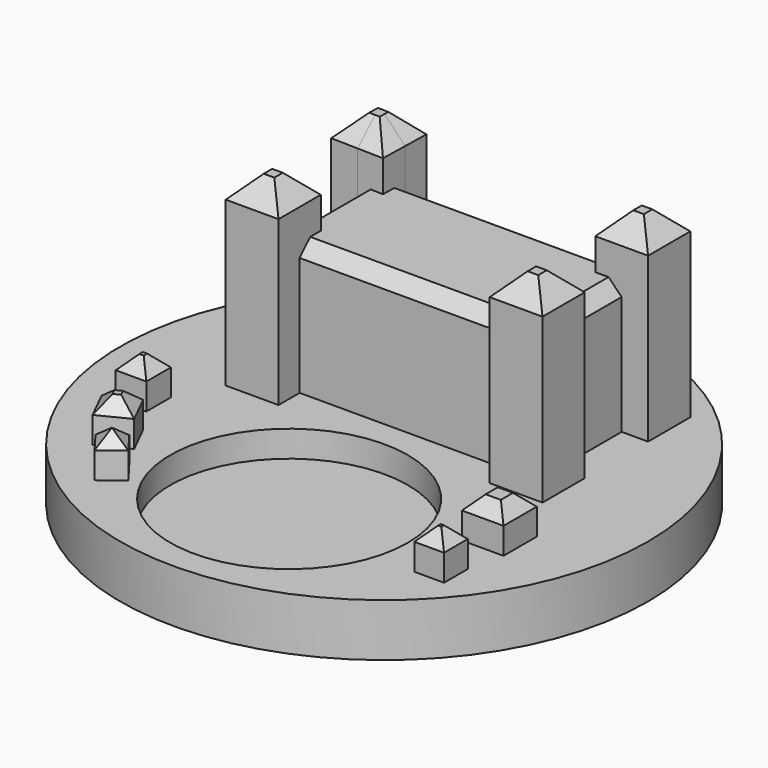
from build123d import *

# Parameters (mm, degrees)
F0_R     = 25.4
F0_W     = 2.9527507722
F0_H     = 2.9527507722
F0_R_2   = 11.43
F0_W_2   = 2.8575006872
F0_H_2   = 2.8575006872
F0_W_3   = 4.0005007759
F0_H_3   = 4.0005007759
F1_DEPTH = 5.08
F2_DEPTH = 2.54
F3_DEPTH = 17.78
F0_W_4   = 2.54
F0_H_4   = 2.54
F0_W_5   = 2.5392780889
F0_H_5   = 2.5392780889
F4_DEPTH = 22.86
F5_DEPTH = 8.89
F6_SIZE  = 1.26999
F7_SIZE  = 2.032
F8_SIZE  = 1.27


# Not quite as in the source:
# - a fillet or chamfer is up to 0.001 mm smaller than in the source, because OpenCascade refuses the exact size


with BuildPart() as f1:
    # F0 (on Top) → F1 (new body)
    with BuildSketch(Plane.XY):
        Circle(F0_R)
        Polygon((-14.8460203377, -16.160586299), (-12.8199555069, -14.6287046778), (-11.2880738857, -16.6547695086), (-13.3141387165, -18.1866511298), align=None, mode=Mode.SUBTRACT)
        Polygon((-17.0199228451, -13.7883033603), (-18.4486722574, -10.9308026731), (-15.5911715701, -9.5020532608), (-14.1624221578, -12.359553948), align=None, mode=Mode.SUBTRACT)
        with Locations((-18.734421581, -5.5491779931)):
            Rectangle(F0_W, F0_H, mode=Mode.SUBTRACT)
        with Locations((0, -11.43)):
            Circle(F0_R_2, mode=Mode.SUBTRACT)
        with Locations((16.1819914356, -13.3789330721)):
            Rectangle(F0_W_2, F0_H_2, mode=Mode.SUBTRACT)
        with Locations((16.3652040064, -6.5969279967)):
            Rectangle(F0_W_3, F0_H_3, mode=Mode.SUBTRACT)
        Polygon((-10.1001541496, 17.7187103274), (-10.1592772274, 15.24), (10.1607219111, 15.24), (10.1607219111, 17.7792780889), (15.2392780889, 17.7792780889), (15.2392780889, 12.7007219111), (12.7, 12.7007219111), (12.7, 5.08), (15.24, 5.08), (15.24, 0), (10.16, 0), (10.16, 2.54), (-10.16, 2.54), (-10.16, 0), (-15.24, 0), (-15.24, 5.08), (-12.7, 5.08), (-12.7, 12.6992772274), (-15.2998458504, 12.7612896726), (-15.1787103274, 17.8398458504), align=None, mode=Mode.SUBTRACT)
    extrude(amount=F1_DEPTH)

    # F0 (on Top) → F2 (join)
    with BuildSketch(Plane.XY):
        with Locations((0, -11.43)):
            Circle(F0_R_2)
    extrude(amount=F2_DEPTH)

    # F0 (on Top) → F3 (join)
    with BuildSketch(Plane.XY):
        Polygon((10.1607219111, 15.24), (-10.1592772274, 15.24), (-10.2212896726, 12.6401541496), (-12.7, 12.6992772274), (-12.7, 5.08), (-10.16, 5.08), (-10.16, 2.54), (10.16, 2.54), (10.16, 5.08), (12.7, 5.08), (12.7, 12.7007219111), (10.1607219111, 12.7007219111), align=None)
    extrude(amount=F3_DEPTH)

    # F0 (on Top) → F4 (join)
    with BuildSketch(Plane.XY):
        Polygon((-10.1592772274, 15.24), (-12.7, 15.24), (-12.7, 12.6992772274), (-10.2212896726, 12.6401541496), align=None)
        Polygon((-12.7, 12.6992772274), (-12.7, 15.24), (-10.1592772274, 15.24), (-10.1001541496, 17.7187103274), (-15.1787103274, 17.8398458504), (-15.2998458504, 12.7612896726), align=None)
        with Locations((-11.43, 3.81)):
            Rectangle(F0_W_4, F0_H_4)
        Polygon((-12.7, 2.54), (-12.7, 5.08), (-15.24, 5.08), (-15.24, 0), (-10.16, 0), (-10.16, 2.54), align=None)
        with Locations((11.4303609556, 13.9703609556)):
            Rectangle(F0_W_5, F0_H_5)
        Polygon((10.1607219111, 17.7792780889), (10.1607219111, 15.24), (12.7, 15.24), (12.7, 12.7007219111), (15.2392780889, 12.7007219111), (15.2392780889, 17.7792780889), align=None)
        with Locations((11.43, 3.81)):
            Rectangle(F0_W_4, F0_H_4)
        Polygon((15.24, 5.08), (12.7, 5.08), (12.7, 2.54), (10.16, 2.54), (10.16, 0), (15.24, 0), align=None)
    extrude(amount=F4_DEPTH)

    # F0 (on Top) → F5 (join)
    with BuildSketch(Plane.XY):
        with Locations((-18.734421581, -5.5491779931)):
            Rectangle(F0_W, F0_H)
        Polygon((-15.5911715701, -9.5020532608), (-18.4486722574, -10.9308026731), (-17.0199228451, -13.7883033603), (-14.1624221578, -12.359553948), align=None)
        Polygon((-11.2880738857, -16.6547695086), (-12.8199555069, -14.6287046778), (-14.8460203377, -16.160586299), (-13.3141387165, -18.1866511298), align=None)
        with Locations((16.3652040064, -6.5969279967)):
            Rectangle(F0_W_3, F0_H_3)
        with Locations((16.1819914356, -13.3789330721)):
            Rectangle(F0_W_2, F0_H_2)
    extrude(amount=F5_DEPTH)

    # F6 (size 1.27 in the source; OpenCascade refuses exactly that, so slightly less here)
    f6_edges = [f1.edges().sort_by_distance(p)[0] for p in [
        (-18.734422, -4.072803, 8.89),
        (-20.210797, -5.549178, 8.89),
        (-18.734422, -7.025553, 8.89),
        (-17.258046, -5.549178, 8.89),
        (-17.019922, -10.216428, 8.89),
        (-17.734298, -12.359553, 8.89),
        (-15.591173, -13.073929, 8.89),
        (-14.876797, -10.930804, 8.89),
        (-12.301106, -17.42071, 8.89),
        (-12.054015, -15.641737, 8.89),
        (-13.832988, -15.394645, 8.89),
        (-14.08008, -17.173619, 8.89),
        (16.365204, -4.596678, 8.89),
        (14.364954, -6.596928, 8.89),
        (16.365204, -8.597178, 8.89),
        (18.365454, -6.596928, 8.89),
        (16.181991, -14.807683, 8.89),
        (17.610742, -13.378933, 8.89),
        (16.181991, -11.950183, 8.89),
        (14.753241, -13.378933, 8.89),
    ]]
    chamfer(f6_edges, length=F6_SIZE)

    # F7
    f7_edges = [f1.edges().sort_by_distance(p)[0] for p in [
        (-10.160722, 15.179432, 22.86),
        (-12.639432, 17.779278, 22.86),
        (-15.239278, 15.300568, 22.86),
        (-12.760568, 12.700722, 22.86),
        (-12.7, 5.08, 22.86),
        (-15.24, 2.54, 22.86),
        (-12.7, 0, 22.86),
        (-10.16, 2.54, 22.86),
        (12.7, 12.700722, 22.86),
        (15.239278, 15.24, 22.86),
        (12.7, 17.779278, 22.86),
        (10.160722, 15.24, 22.86),
        (10.16, 2.54, 22.86),
        (12.7, 0, 22.86),
        (15.24, 2.54, 22.86),
        (12.7, 5.08, 22.86),
    ]]
    chamfer(f7_edges, length=F7_SIZE)

    # F8
    f8_edges = [f1.edges().sort_by_distance(p)[0] for p in [
        (0, 2.54, 17.78),
        (0.000722, 15.24, 17.78),
        (-12.7, 8.889639, 17.78),
        (12.7, 8.890361, 17.78),
    ]]
    chamfer(f8_edges, length=F8_SIZE)


solid = f1.part
